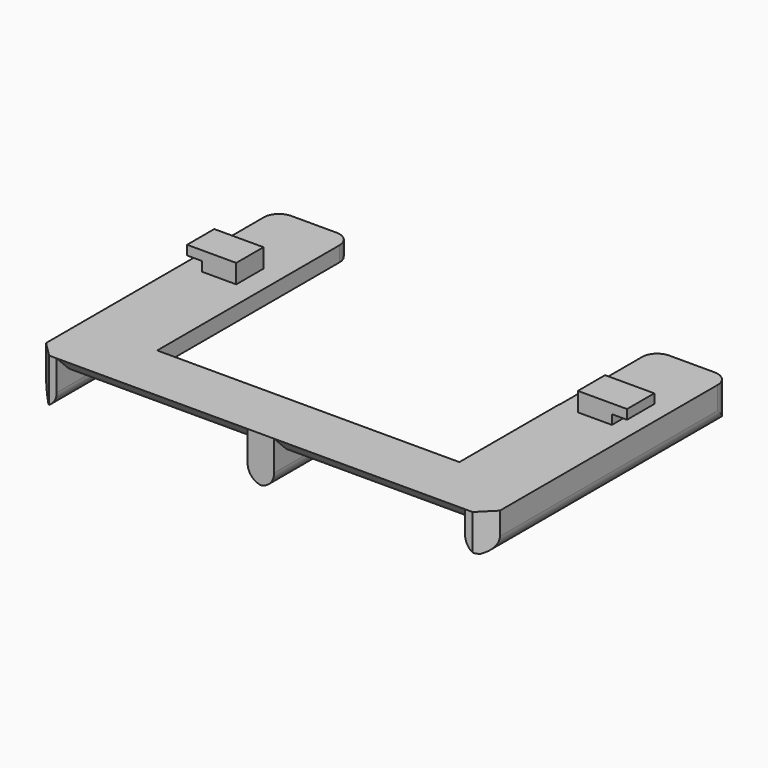
from build123d import *

# Parameters (mm, degrees)
F0_W          = 152.4
F0_H          = 101.6
F1_DEPTH      = 5.08
F2_W          = 7.62
F2_H          = 101.6
F3_DEPTH      = 10.16
F4_T1_DEPTH   = 127
F5_W          = 7.62
F5_H          = 101.6
F6_DEPTH      = 7.62
F7_T1_DEPTH   = 127
F8_W          = 8.89
F8_H          = 101.6
F9_DEPTH      = 10.16
F10_T1_DEPTH  = 127
F11_W         = 101.6
F11_H         = 43.9456890713
F12_DEPTH     = 25.4
F13_T1_DEPTH  = 5.08
F13_T3_DEPTH  = 30.48
F13_T5_DEPTH  = 35.56
F13_T7_DEPTH  = 33.02
F14_T1_DEPTH  = 36.2882991577
F14_T3_DEPTH  = 33.7482991577
F14_T5_DEPTH  = 64.1381350342
F14_T7_DEPTH  = 64.1318649658
F14_T12_DEPTH = 90.2664341919
F14_T17_DEPTH = 90.2601641236
F15_W         = 11.43
F15_H         = 11.43
F16_DEPTH     = 6.35
F17_W         = 11.43
F17_H         = 11.43
F18_DEPTH     = 6.35
F19_W         = 11.43
F19_H         = 3.175
F20_DEPTH     = 5.08
F21_W         = 11.43
F21_H         = 3.175
F22_DEPTH     = 5.08
F23_W         = 101.4830252707
F23_H         = 42.7652306713
F24_DEPTH     = 25.4


# Not quite as in the source:
# - a fillet or chamfer that OpenCascade refuses, or shapes differently, is made with other operations: its cross-section is extruded or revolved along the edge and cut away or added


with BuildPart() as f1:
    # F0 (on Top) → F1 (new body)
    with BuildSketch(Plane.XY):
        Rectangle(F0_W, F0_H)
    extrude(amount=F1_DEPTH)

    # F2 (on face) → F3 (join)
    with BuildSketch(Plane(origin=(0, 0, 0), x_dir=(1, 0, 0), z_dir=(0, 0, -1))):
        with Locations((-72.39, 0)):
            Rectangle(F2_W, F2_H)
    extrude(amount=F3_DEPTH)

    # F4: fillet of radius 5.08 on 2 edges, made by hand

    # F4_s2 → F4_t1 (cut)
    with BuildSketch(Plane.XZ.offset(-63.5)):
        with BuildLine():
            ThreePointArc((-71.12, -10.16), (-74.7121024484, -8.6721024484), (-76.2, -5.08))
            Line((-76.2, -5.08), (-76.2, -10.16))
            Line((-76.2, -10.16), (-71.12, -10.16))
        make_face()
        with BuildLine():
            ThreePointArc((-68.58, -5.08), (-70.0678975516, -8.6721024484), (-73.66, -10.16))
            Line((-73.66, -10.16), (-68.58, -10.16))
            Line((-68.58, -10.16), (-68.58, -5.08))
        make_face()
    extrude(amount=F4_T1_DEPTH, mode=Mode.SUBTRACT)

    # F5 (on face) → F6 (join)
    with BuildSketch(Plane(origin=(0, 0, 0), x_dir=(1, 0, 0), z_dir=(0, 0, -1))):
        with Locations((72.39, 0)):
            Rectangle(F5_W, F5_H)
    extrude(amount=F6_DEPTH)

    # F7: fillet of radius 5.08 on 2 edges, made by hand

    # F7_s2 → F7_t1 (cut)
    with BuildSketch(Plane.XZ.offset(-63.5)):
        with BuildLine():
            ThreePointArc((76.2, -2.54), (74.7121024484, -6.1321024484), (71.12, -7.62))
            Line((71.12, -7.62), (76.2, -7.62))
            Line((76.2, -7.62), (76.2, -2.54))
        make_face()
        with BuildLine():
            ThreePointArc((73.66, -7.62), (70.0678975516, -6.1321024484), (68.58, -2.54))
            Line((68.58, -2.54), (68.58, -7.62))
            Line((68.58, -7.62), (73.66, -7.62))
        make_face()
    extrude(amount=F7_T1_DEPTH, mode=Mode.SUBTRACT)

    # F8 (on face) → F9 (join)
    with BuildSketch(Plane(origin=(0, 0, 0), x_dir=(1, 0, 0), z_dir=(0, 0, -1))):
        with Locations((-0.0031350342, 0)):
            Rectangle(F8_W, F8_H)
    extrude(amount=F9_DEPTH)

    # F10: fillet of radius 5.08 on 2 edges, made by hand

    # F10_s2 → F10_t1 (cut)
    with BuildSketch(Plane.XZ.offset(-63.5)):
        with BuildLine():
            ThreePointArc((-4.4481350342, -5.08), (-2.9602374826, -8.6721024484), (0.6318649658, -10.16))
            Line((0.6318649658, -10.16), (-4.4481350342, -10.16))
            Line((-4.4481350342, -10.16), (-4.4481350342, -5.08))
        make_face()
        with BuildLine():
            ThreePointArc((4.4418649658, -5.08), (2.9539674142, -8.6721024484), (-0.6381350342, -10.16))
            Line((-0.6381350342, -10.16), (4.4418649658, -10.16))
            Line((4.4418649658, -10.16), (4.4418649658, -5.08))
        make_face()
    extrude(amount=F10_T1_DEPTH, mode=Mode.SUBTRACT)

    # F11 (on face) → F12 (cut)
    with BuildSketch(Plane.XY.offset(5.08)):
        with Locations((0, 28.8271554643)):
            Rectangle(F11_W, F11_H)
    extrude(amount=-F12_DEPTH, mode=Mode.SUBTRACT)

    # F13: fillet of radius 5.08 on 5 edges, made by hand

    # F13_s2 → F13_t1 (join)
    with BuildSketch(Plane.XY):
        with BuildLine():
            ThreePointArc((50.8, 11.9343109287), (49.3121024484, 8.3422084803), (45.72, 6.8543109287))
            Line((45.72, 6.8543109287), (50.8, 6.8543109287))
            Line((50.8, 6.8543109287), (50.8, 11.9343109287))
        make_face()
    extrude(amount=F13_T1_DEPTH)

    # F13_s4 → F13_t3 (cut)
    with BuildSketch(Plane.XY.offset(-12.7)):
        with BuildLine():
            ThreePointArc((-55.88, 50.8), (-52.2878975516, 49.3121024484), (-50.8, 45.72))
            Line((-50.8, 45.72), (-50.8, 50.8))
            Line((-50.8, 50.8), (-55.88, 50.8))
        make_face()
        with BuildLine():
            ThreePointArc((55.88, 50.8), (52.2878975516, 49.3121024484), (50.8, 45.72))
            Line((50.8, 45.72), (50.8, 50.8))
            Line((50.8, 50.8), (55.88, 50.8))
        make_face()
    extrude(amount=F13_T3_DEPTH, mode=Mode.SUBTRACT)

    # F13_s6 → F13_t5 (cut)
    with BuildSketch(Plane.XY.offset(-17.78)):
        with BuildLine():
            ThreePointArc((-76.2, 45.72), (-74.7121024484, 49.3121024484), (-71.12, 50.8))
            Line((-71.12, 50.8), (-76.2, 50.8))
            Line((-76.2, 50.8), (-76.2, 45.72))
        make_face()
    extrude(amount=F13_T5_DEPTH, mode=Mode.SUBTRACT)

    # F13_s8 → F13_t7 (cut)
    with BuildSketch(Plane.XY.offset(-15.24)):
        with BuildLine():
            ThreePointArc((71.12, 50.8), (74.7121024484, 49.3121024484), (76.2, 45.72))
            Line((76.2, 45.72), (76.2, 50.8))
            Line((76.2, 50.8), (71.12, 50.8))
        make_face()
    extrude(amount=F13_T7_DEPTH, mode=Mode.SUBTRACT)

    # F14: chamfer of 5.08 on 4 edges, made by hand

    # F14_s2 → F14_t1 (cut)
    with BuildSketch(Plane.XY.offset(-18.1441495789)):
        Polygon((-71.12, -50.8), (-76.2, -45.72), (-76.2, -50.8), align=None)
    extrude(amount=F14_T1_DEPTH, mode=Mode.SUBTRACT)

    # F14_s4 → F14_t3 (cut)
    with BuildSketch(Plane.XY.offset(-15.6041495789)):
        Polygon((71.12, -50.8), (76.2, -45.72), (76.2, -50.8), align=None)
    extrude(amount=F14_T3_DEPTH, mode=Mode.SUBTRACT)

    # F14_s6 → F14_t5 (cut)
    with BuildSketch(Plane.YZ.offset(4.4418649658)):
        Polygon((-45.72, 0), (-50.8, 5.08), (-50.8, 0), align=None)
    extrude(amount=F14_T5_DEPTH, mode=Mode.SUBTRACT)

    # F14_s8 → F14_t7 (cut)
    with BuildSketch(Plane.YZ.offset(-68.58)):
        Polygon((-50.8, 5.08), (-45.72, 0), (-50.8, 0), align=None)
    extrude(amount=F14_T7_DEPTH, mode=Mode.SUBTRACT)


with BuildPart() as f14_tool10:
    # F14_s11 → F14_t12 (new body)
    with BuildSketch(Plane.YZ.offset(-8.622284613)):
        Polygon((-45.72, 0), (-50.8, 5.08), (-50.8, 0), align=None)
    extrude(amount=F14_T12_DEPTH)

    split(bisect_by=Plane.YZ.offset(-4.4481350342), keep=Keep.BOTTOM)


with BuildPart() as f1_1:
    add(f1.part)

    # F14_t9: cut F14_tool10
    add(f14_tool10.part, mode=Mode.SUBTRACT)


with BuildPart() as f14_tool15:
    # F14_s16 → F14_t17 (new body)
    with BuildSketch(Plane.YZ.offset(-81.6441495789)):
        Polygon((-50.8, 5.08), (-45.72, 0), (-50.8, 0), align=None)
    extrude(amount=F14_T17_DEPTH)

    split(bisect_by=Plane.YZ.offset(4.4418649658), keep=Keep.TOP)


with BuildPart() as f1_2:
    add(f1_1.part)

    # F14_t14: cut F14_tool15
    add(f14_tool15.part, mode=Mode.SUBTRACT)

    # F15 (on face) → F16 (join)
    with BuildSketch(Plane.XY.offset(5.08)):
        with Locations((63.0153976381, 16.3576488795)):
            Rectangle(F15_W, F15_H)
    extrude(amount=F16_DEPTH)

    # F17 (on face) → F18 (join)
    with BuildSketch(Plane.XY.offset(5.08)):
        with Locations((-63.7673679739, 17.1340169625)):
            Rectangle(F17_W, F17_H)
    extrude(amount=F18_DEPTH)

    # F19 (on face) → F20 (join)
    with BuildSketch(Plane(origin=(-69.4823679739, 0, 0), x_dir=(0, -1, 0), z_dir=(-1, 0, 0))):
        with Locations((-17.1340169625, 9.8425)):
            Rectangle(F19_W, F19_H)
    extrude(amount=F20_DEPTH)

    # F21 (on face) → F22 (join)
    with BuildSketch(Plane.YZ.offset(68.7303976381)):
        with Locations((16.3576488795, 9.8425)):
            Rectangle(F21_W, F21_H)
    extrude(amount=F22_DEPTH)

    # F23 (on face) → F24 (cut)
    with BuildSketch(Plane.XY.offset(5.08)):
        with Locations((-0.0584873646, -9.448304407)):
            Rectangle(F23_W, F23_H)
    extrude(amount=-F24_DEPTH, mode=Mode.SUBTRACT)


solid = f1_2.part
